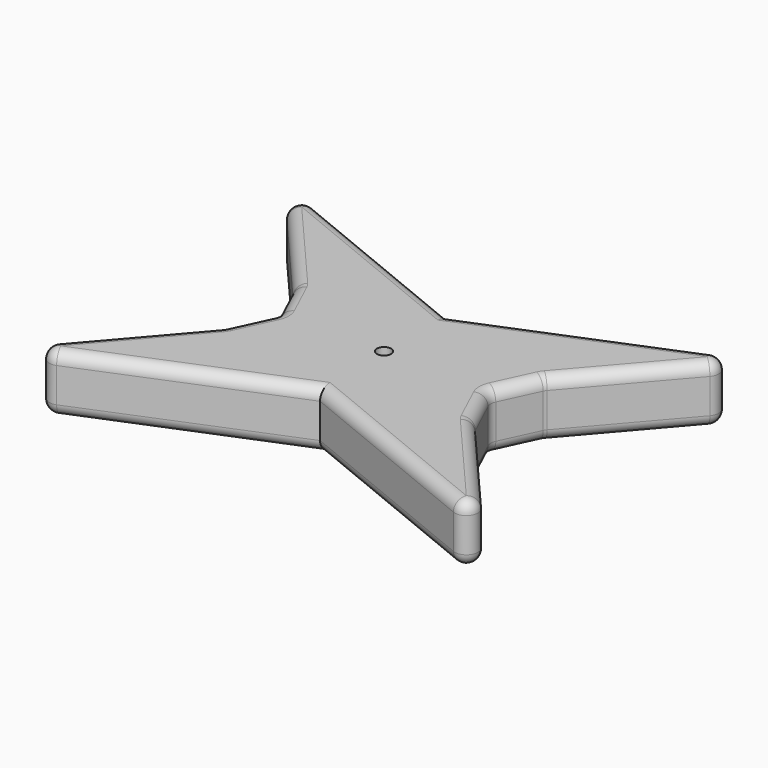
from build123d import *

# Parameters (mm, degrees)
F2_DEPTH = 25.4
F3_F1_R  = 5.08
F3_F2_R  = 5.08
F6_D     = 6.35


# Not quite as in the source:
# - the program builds the solid bodies; features that only make, move or delete a surface that nothing else refers to are left out


with BuildPart() as f2:
    # F1 (on Top) → F2 (new body)
    with BuildSketch(Plane.XY):
        Polygon((-107.0532500744, -79.1042298079), (0, -35.2327227592), (107.0532500744, -79.1042298079), (55.5592626333, -19.3102359772), (46.5817004442, 0), (55.5592626333, 19.3102359772), (107.0532500744, 79.1042298079), (0, 35.2327227592), (-107.0532500744, 79.1042298079), (-55.5592626333, 19.3102359772), (-46.5817004442, 0), (-55.5592626333, -19.3102359772), align=None)
    extrude(amount=F2_DEPTH)

    # F3: fillet of radius 5.08 on 32 edges, made by hand

    # F3_f1
    f3_f1_edges = [f2.edges().sort_by_distance(p)[0] for p in [
        (-55.5592626333, -19.3102359772, 12.7),
        (-46.5817004442, 0, 12.7),
        (-55.5592626333, 19.3102359772, 12.7),
        (55.5592626333, -19.3102359772, 12.7),
        (46.5817004442, 0, 12.7),
        (55.5592626333, 19.3102359772, 12.7),
    ]]
    fillet(f3_f1_edges, radius=F3_F1_R)

    # F3_f2
    f3_f2_edges = [f2.edges().sort_by_distance(p)[0] for p in [
        (53.5266250372, 57.1684762836, 25.4),
        (53.5266250372, 57.1684762836, 0),
        (107.0532500744, 79.1042298079, 12.7),
        (81.5362590314, 49.4743083195, 25.4),
        (51.4197227557, 10.4063163842, 25.4),
        (51.4197227557, -10.4063163842, 25.4),
        (81.5362590314, -49.4743083195, 25.4),
        (107.0532500744, -79.1042298079, 12.7),
        (53.5266250372, -57.1684762836, 0),
        (53.5266250372, -57.1684762836, 25.4),
        (-81.5362590314, 49.4743083195, 25.4),
        (-53.5266250372, 57.1684762836, 25.4),
        (-51.4197227557, 10.4063163842, 25.4),
        (-51.4197227557, -10.4063163842, 25.4),
        (-81.5362590314, -49.4743083195, 25.4),
        (-53.5266250372, 57.1684762836, 0),
        (-107.0532500744, 79.1042298079, 12.7),
        (-81.5362590314, 49.4743083195, 0),
        (-53.5266250372, -57.1684762836, 0),
        (-107.0532500744, -79.1042298079, 12.7),
        (-53.5266250372, -57.1684762836, 25.4),
        (81.5362590314, -49.4743083195, 0),
        (51.4197227557, -10.4063163842, 0),
        (51.4197227557, 10.4063163842, 0),
        (-51.4197227557, 10.4063163842, 0),
        (-51.4197227557, -10.4063163842, 0),
        (-47.1038678133, 0, 0),
        (-55.6001625442, -19.2838429205, 0),
        (-55.6001625442, 19.2838429205, 0),
        (47.1038678133, 0, 0),
        (55.6001625442, 19.2838429205, 0),
        (55.6001625442, -19.2838429205, 0),
        (-55.6001625442, -19.2838429205, 25.4),
        (-47.1038678133, 0, 25.4),
        (-55.6001625442, 19.2838429205, 25.4),
        (55.6001625442, -19.2838429205, 25.4),
        (47.1038678133, 0, 25.4),
        (55.6001625442, 19.2838429205, 25.4),
    ]]
    fillet(f3_f2_edges, radius=F3_F2_R)

    # F6 (through all)
    with Locations(Plane.XY.offset(25.4)):
        with Locations((0, 0)):
            Hole(F6_D / 2)


solid = f2.part
